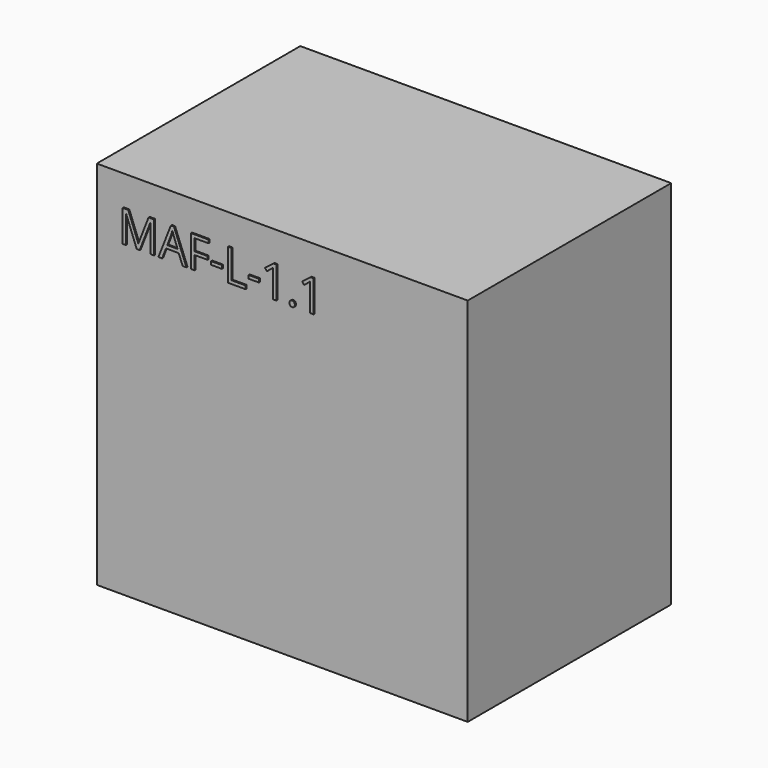
from build123d import *

# Parameters (mm, degrees)
F0_W         = 1778
F0_H         = 965.2
F1_DEPTH     = 1778
F2_TEXT_SIZE = 212.6299672657
F3_DEPTH     = 6.35
F4_DEPTH     = 254


# Not quite as in the source:
# - Text() gives the source's letters only with a copy of the font that has no kerning and outlines rounded to 1/6400 em; it was checked with that copy


with BuildPart() as f1:
    # F0 (on Top) → F1 (new body)
    with BuildSketch(Plane.XY):
        with Locations((889, 482.6)):
            Rectangle(F0_W, F0_H)
    extrude(amount=F1_DEPTH)

    # F2 (on face) → F3 (join)
    with BuildSketch(Plane.XZ):
        with Locations((108.3469837904, 1483.6558103561)):
            Text('MAF-L-1.1', F2_TEXT_SIZE, font='Open Sans', text_align=(TextAlign.LEFT, TextAlign.BOTTOM))
    extrude(amount=F3_DEPTH)

    # F4 (add): a face of the model
    f4_faces = [f1.faces().sort_by_distance(p)[0] for p in [
        (889, 965.2, 889),
    ]]
    extrude(f4_faces, amount=F4_DEPTH)


solid = f1.part
